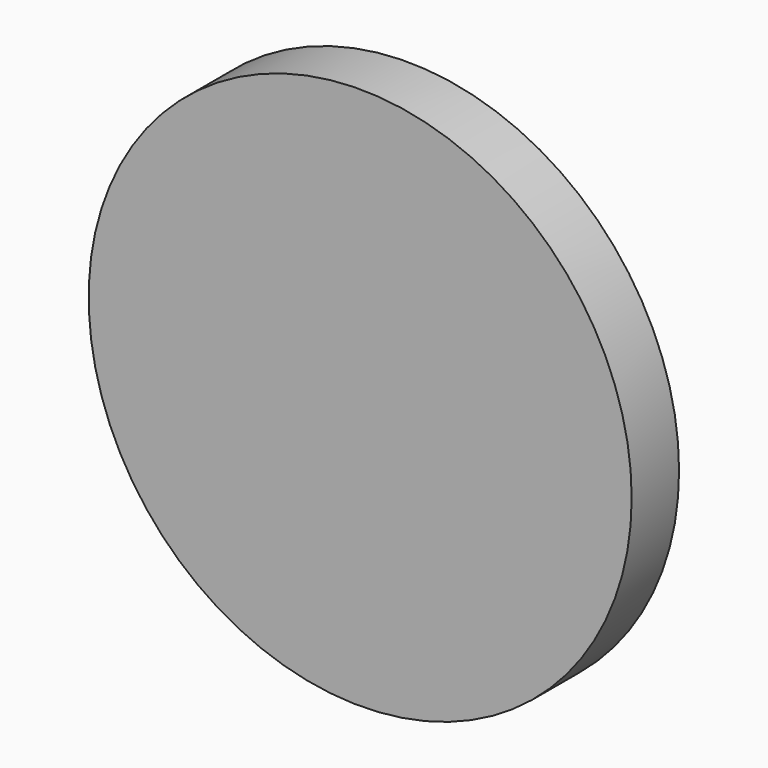
from build123d import *

# Parameters (mm, degrees)
F0_R         = 27.5
F1_DEPTH     = 6
F2_R         = 22.5
F3_DEPTH     = 4
F4_R         = 2.5
F4_R_2       = 4
F4_TEXT_SIZE = 23.5274091311
F5_DEPTH     = 4


# Not quite as in the source:
# - Text() gives the source's letters only with a copy of the font that has no kerning and outlines rounded to 1/6400 em; it was checked with that copy


with BuildPart() as f1:
    # F0 (on Front) → F1 (new body)
    with BuildSketch(Plane.XZ):
        Circle(F0_R)
    extrude(amount=F1_DEPTH)

    # F2 (on Front) → F3 (cut)
    with BuildSketch(Plane.XZ):
        Circle(F2_R)
    extrude(amount=F3_DEPTH, mode=Mode.SUBTRACT)

    # F4 (on face) → F5 (join, through all)
    with BuildSketch(Plane(origin=(0, -4, 0), x_dir=(-1, 0, 0), z_dir=(0, 1, 0))):
        with Locations((-14.446338135, 8.5604224345)):
            Circle(F4_R)
        with Locations((0, 15.0895873117)):
            Circle(F4_R_2)
        with Locations((13.8154209236, 8.5604224345)):
            Circle(F4_R)
        with Locations((-15.8810019493, -12.2510588262)):
            Text('AC', F4_TEXT_SIZE, font='Open Sans', font_style=FontStyle.BOLD, text_align=(TextAlign.LEFT, TextAlign.BOTTOM))
    extrude(amount=F5_DEPTH)


solid = f1.part
